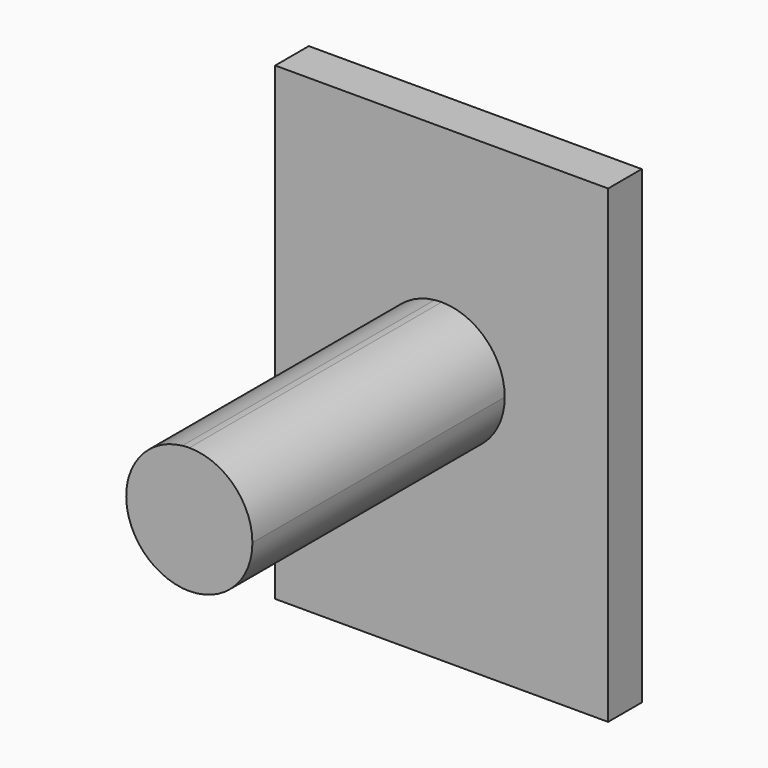
from build123d import *

# Parameters (mm, degrees)
F1_DEPTH = 12
F3_DEPTH = 90


with BuildPart() as f1:
    # F0 (on Front) → F1 (new body)
    with BuildSketch(Plane.XZ):
        Polygon((47.5, -67), (47.5, 0), (47.5, 67), (0, 67), (-47.5, 67), (-47.5, -67), align=None)
    extrude(amount=F1_DEPTH)

    # F2 (on face) → F3 (join)
    with BuildSketch(Plane.XZ.offset(12)):
        with BuildLine():
            Line((0, 5), (0, 0))
            Line((0, 0), (-4.8013158464, 0))
            ThreePointArc((-4.8013158464, 0), (-1.2386876382, -6.0708472044), (0, -13))
            ThreePointArc((0, -13), (12.7279220614, -7.7279220614), (18, 5))
            ThreePointArc((18, 5), (12.7279220614, 17.7279220614), (0, 23))
            Line((0, 23), (0, 5))
        make_face()
        with BuildLine():
            Line((-4.8013158464, 0), (0, 0))
            Line((0, 0), (0, 5))
            Line((0, 5), (0, 23))
            ThreePointArc((0, 23), (-5.397234005, 11.476680806), (-17.7049180328, 8.2459016393))
            ThreePointArc((-17.7049180328, 8.2459016393), (-17.8156486606, 7.5695647107), (-17.9005524862, 6.8895027624))
            ThreePointArc((-17.9005524862, 6.8895027624), (-10.6901851858, 4.7010550004), (-4.8013158464, 0))
        make_face()
        with BuildLine():
            ThreePointArc((0, -13), (-1.2386876382, -6.0708472044), (-4.8013158464, 0))
            Line((-4.8013158464, 0), (-7.550100402, 0))
            ThreePointArc((-7.550100402, 0), (-3.4675400893, -5.881167982), (-2.0003453113, -12.8885052096))
            ThreePointArc((-2.0003453113, -12.8885052096), (-1.0017250687, -12.9721046872), (0, -13))
        make_face()
        with BuildLine():
            Line((-7.550100402, 0), (-4.8013158464, 0))
            ThreePointArc((-4.8013158464, 0), (-10.6901851858, 4.7010550004), (-17.9005524862, 6.8895027624))
            ThreePointArc((-17.9005524862, 6.8895027624), (-17.9779647514, 5.8903838491), (-17.9996546887, 4.8885052096))
            ThreePointArc((-17.9996546887, 4.8885052096), (-12.3726305137, 3.3040864423), (-7.550100402, 0))
        make_face()
        with BuildLine():
            ThreePointArc((-2.0003453113, -12.8885052096), (-3.4675400893, -5.881167982), (-7.550100402, 0))
            Line((-7.550100402, 0), (-17.2916164658, 0))
            ThreePointArc((-17.2916164658, 0), (-11.6005749399, -8.76323585), (-2.0003453113, -12.8885052096))
        make_face()
        with BuildLine():
            Line((-17.2916164658, 0), (-7.550100402, 0))
            ThreePointArc((-7.550100402, 0), (-12.3726305137, 3.3040864423), (-17.9996546887, 4.8885052096))
            ThreePointArc((-17.9996546887, 4.8885052096), (-17.8141187186, 2.4198499502), (-17.2916164658, 0))
        make_face()
        with BuildLine():
            ThreePointArc((-17.7049180328, 8.2459016393), (-5.397234005, 11.476680806), (0, 23))
            ThreePointArc((0, 23), (-1.0017918512, 22.9721009647), (-2.0004782551, 22.888490343))
            ThreePointArc((-2.0004782551, 22.888490343), (-6.6776028044, 13.0131233652), (-17.2344944225, 10.1934768701))
            ThreePointArc((-17.2344944225, 10.1934768701), (-17.4968253692, 9.2262396998), (-17.7049180328, 8.2459016393))
        make_face()
        with BuildLine():
            ThreePointArc((-17.2344944225, 10.1934768701), (-6.6776028044, 13.0131233652), (-2.0004782551, 22.888490343))
            ThreePointArc((-2.0004782551, 22.888490343), (-11.523319194, 18.8279830328), (-17.2344944225, 10.1934768701))
        make_face()
    extrude(amount=F3_DEPTH)


solid = f1.part
